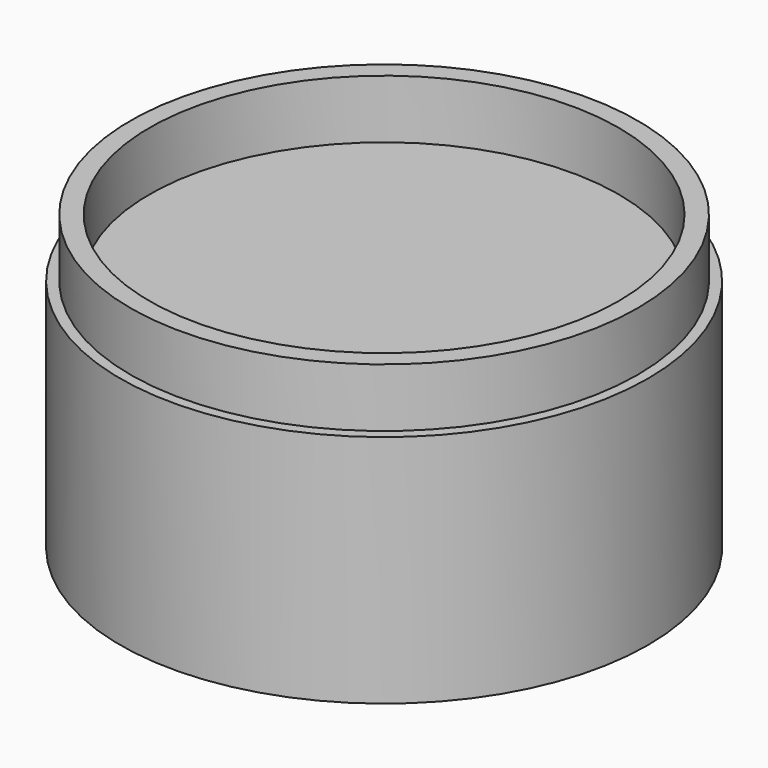
from build123d import *

# Parameters (mm, degrees)
F0_R     = 45
F1_DEPTH = 40
F2_R     = 43.25
F3_DEPTH = 10
F4_R     = 40
F5_DEPTH = 40


with BuildPart() as f1:
    # F0 (on Top) → F1 (new body)
    with BuildSketch(Plane.XY):
        Circle(F0_R)
    extrude(amount=F1_DEPTH)


with BuildPart() as f3:
    # F2 (on face) → F3 (new body)
    with BuildSketch(Plane.XY.offset(40)):
        Circle(F2_R)
    extrude(amount=F3_DEPTH)

    # F4 (on face) → F5 (cut)
    with BuildSketch(Plane.XY.offset(50)):
        Circle(F4_R)
    extrude(amount=-F5_DEPTH, mode=Mode.SUBTRACT)


solid = Compound([f1.part, f3.part])
